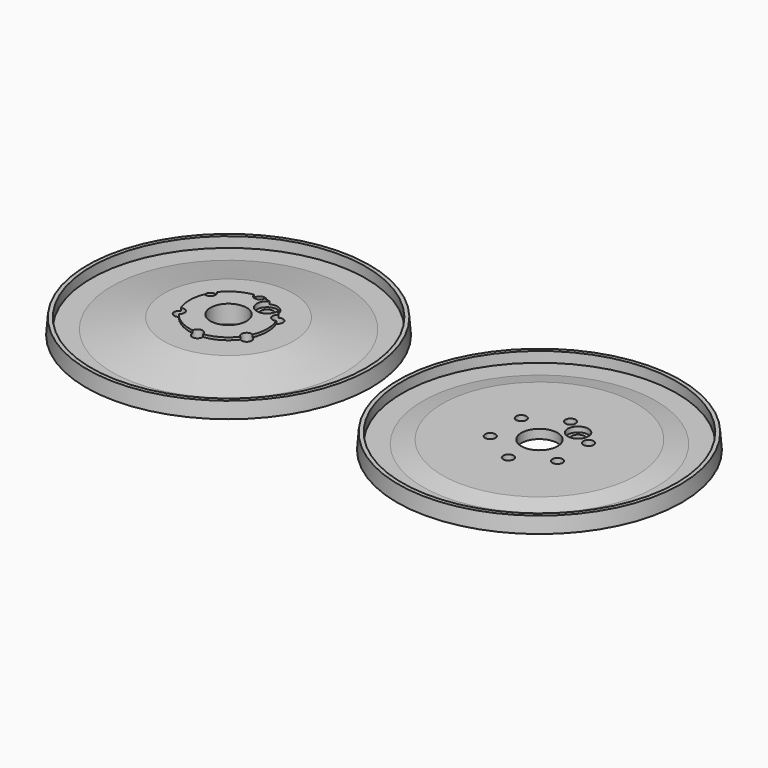
from build123d import *

# Parameters (mm, degrees)
F3_D           = 5
F3_CBORE_D     = 8
F3_CBORE_DEPTH = 2
F4_D           = 4
F5_D           = 14
F7_R           = 50
F7_R_2         = 2.5
F8_DEPTH       = 3.5
F9_D           = 5
F9_START       = 3.5
F9_CBORE_D     = 8
F9_CBORE_DEPTH = 2


with BuildPart() as f1:
    # F0 (on Front) → F1 (revolve)
    with BuildSketch(Plane.XZ):
        Polygon((0, 7), (0, 0), (55, 0), (54.5, 6), (53, 6), (53, 2), (45, 2), (25, 6), (15, 6), (15, 7), align=None)
    revolve(axis=Axis((0, 0, 0), (0, 0, -1)))

    # F3 (through all)
    with Locations(Plane.XY.offset(7)):
        with Locations((6.25, 10.8253175473)):
            CounterBoreHole(F3_D / 2, F3_CBORE_D / 2, F3_CBORE_DEPTH)

    # F4 (through all)
    with Locations(Plane.XY.offset(7)):
        with Locations((0, 15), (12.9903810568, 7.5), (12.9903810568, -7.5), (0, -15), (-12.9903810568, -7.5), (-12.9903810568, 7.5)):
            Hole(F4_D / 2)

    # F5 (through all)
    with Locations(Plane.XY.offset(7)):
        with Locations((0, 0)):
            Hole(F5_D / 2)


with BuildPart() as f6_1:
    # F6: copy of F1
    add(f1.part.moved(Location((120, 0, 0))))

    # F7 (on face) → F8 (cut)
    with BuildSketch(Plane.XY.offset(7)):
        with Locations((120, 0)):
            Circle(F7_R)
        with Locations((126.25, 10.8253175473)):
            Circle(F7_R_2, mode=Mode.SUBTRACT)
    extrude(amount=-F8_DEPTH, mode=Mode.SUBTRACT)

    # F9 (through all)
    # its depths count from where the whole tool has entered the part; down to there all is cleared
    with Locations(Plane.XY.offset(7).offset(-F9_START)):
        with Locations((126.25, 10.8253175473)):
            CounterBoreHole(F9_D / 2, F9_CBORE_D / 2, F9_CBORE_DEPTH)


solid = Compound([f1.part, f6_1.part])
